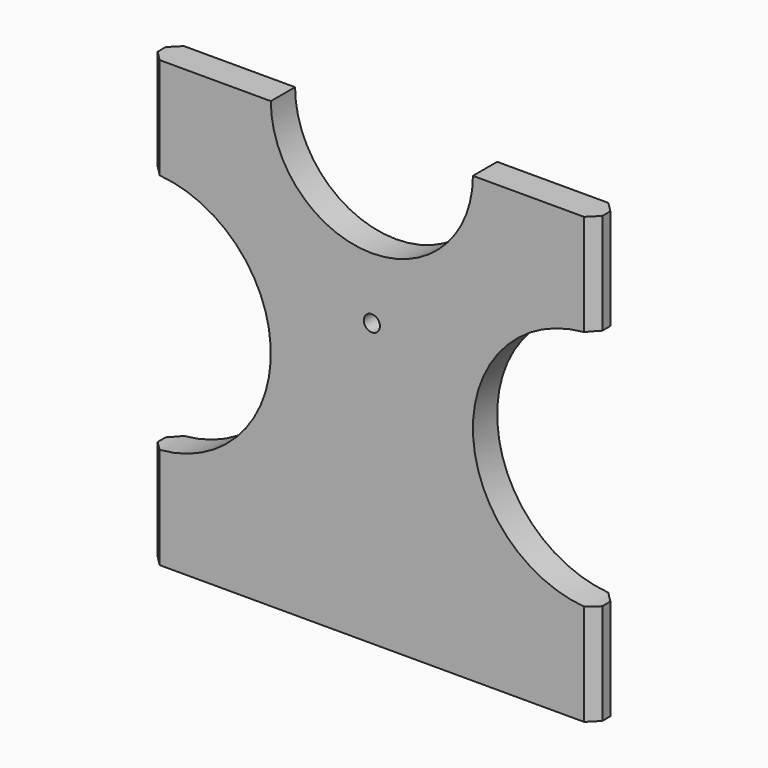
from build123d import *

# Parameters (mm, degrees)
F1_DEPTH = 7.5
F2_SIZE  = 5
F5_R     = 4
F6_DEPTH = 15.001


# Not quite as in the source:
# - two fillets or chamfers of one size are made in one step


with BuildPart() as f1:
    # F0 (on Front) → F1 (new body, symmetric)
    with BuildSketch(Plane.XZ):
        with BuildLine():
            Line((110, 60), (110, 110))
            Line((110, 110), (50, 110))
            ThreePointArc((50, 110), (0, 60), (-50, 110))
            Line((-50, 110), (-110, 110))
            Line((-110, 110), (-110, 60))
            ThreePointArc((-110, 60), (-67.5735931288, 42.4264068712), (-50, 0))
            ThreePointArc((-50, 0), (-67.5735931288, -42.4264068712), (-110, -60))
            Line((-110, -60), (-110, -110))
            Line((-110, -110), (110, -110))
            Line((110, -110), (110, -60))
            ThreePointArc((110, -60), (50, 0), (110, 60))
        make_face()
    extrude(amount=F1_DEPTH, both=True)

    # F2
    f2_edges = [f1.edges().sort_by_distance(p)[0] for p in [
        (-110, 7.5, -85),
        (-110, 7.5, 85),
        (110, 7.5, 85),
        (110, 7.5, -85),
        (110, -7.5, 85),
        (110, -7.5, -85),
        (-110, -7.5, -85),
        (-110, -7.5, 85),
    ]]
    chamfer(f2_edges, length=F2_SIZE)

    # F5 (on face) → F6 (cut, through all)
    with BuildSketch(Plane.XZ.offset(7.5)):
        with Locations((0, 29.5)):
            Circle(F5_R)
    extrude(amount=-F6_DEPTH, mode=Mode.SUBTRACT)


solid = f1.part
